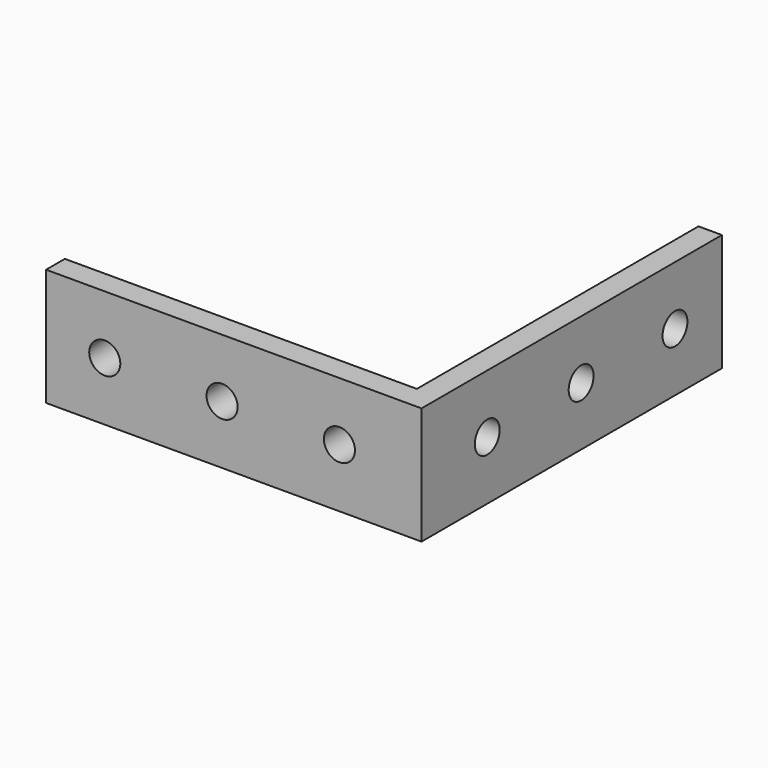
from build123d import *

# Parameters (mm, degrees)
F1_DEPTH  = 20
F2_W      = 9
F2_H      = 20
F2_W_2    = 20
F2_H_2    = 9
F3_DEPTH  = 1.5
F4_W      = 40
F4_H      = 9
F4_W_2    = 9
F4_H_2    = 20
F5_DEPTH  = 1.5
F6_SIZE   = 1.49999
F7_R      = 2.65
F8_DEPTH  = 5.5
F9_R      = 2.65
F10_DEPTH = 5.5


# Not quite as in the source:
# - a fillet or chamfer is up to 0.001 mm smaller than in the source, because OpenCascade refuses the exact size


with BuildPart() as f1:
    # F0 (on Top) → F1 (new body)
    with BuildSketch(Plane.XY):
        Polygon((-64, 0), (0, 0), (0, 64), (-4, 64), (-4, 4), (-64, 4), align=None)
    extrude(amount=F1_DEPTH)

    # F2 (on face) → F3 (join)
    with BuildSketch(Plane(origin=(0, 4, 0), x_dir=(-1, 0, 0), z_dir=(0, 1, 0))):
        with Locations((14, 10)):
            Rectangle(F2_W, F2_H)
        with Locations((34, 10)):
            Rectangle(F2_W, F2_H)
        with Locations((54, 10)):
            Rectangle(F2_W_2, F2_H_2)
    extrude(amount=F3_DEPTH)

    # F4 (on face) → F5 (join)
    with BuildSketch(Plane(origin=(-4, 0, 0), x_dir=(0, -1, 0), z_dir=(-1, 0, 0))):
        with Locations((-44, 10)):
            Rectangle(F4_W, F4_H)
        with Locations((-14, 10)):
            Rectangle(F4_W_2, F4_H_2)
    extrude(amount=F5_DEPTH)

    # F6 (size 1.5 in the source; OpenCascade refuses exactly that, so slightly less here)
    f6_edges = [f1.edges().sort_by_distance(p)[0] for p in [
        (-5.5, 64, 10),
        (-5.5, 44, 14.5),
        (-5.5, 44, 5.5),
        (-5.5, 24, 10),
        (-54, 5.5, 14.5),
        (-54, 5.5, 5.5),
        (-44, 5.5, 10),
        (-64, 5.5, 10),
        (-34, 5.5, 20),
        (-29.5, 5.5, 10),
        (-34, 5.5, 0),
        (-38.5, 5.5, 10),
        (-14, 5.5, 20),
        (-9.5, 5.5, 10),
        (-14, 5.5, 0),
        (-18.5, 5.5, 10),
        (-5.5, 9.5, 10),
        (-5.5, 14, 20),
        (-5.5, 18.5, 10),
        (-5.5, 14, 0),
    ]]
    chamfer(f6_edges, length=F6_SIZE)

    # F7 (on face) → F8 (cut, through all)
    with BuildSketch(Plane(origin=(0, 5.5, 0), x_dir=(-1, 0, 0), z_dir=(0, 1, 0))):
        with Locations((14, 10)):
            Circle(F7_R)
        with Locations((34, 10)):
            Circle(F7_R)
        with Locations((54, 10)):
            Circle(F7_R)
    extrude(amount=-F8_DEPTH, mode=Mode.SUBTRACT)

    # F9 (on face) → F10 (cut, through all)
    with BuildSketch(Plane(origin=(-5.5, 0, 0), x_dir=(0, -1, 0), z_dir=(-1, 0, 0))):
        with Locations((-54, 10)):
            Circle(F9_R)
        with Locations((-34, 10)):
            Circle(F9_R)
        with Locations((-14, 10)):
            Circle(F9_R)
    extrude(amount=-F10_DEPTH, mode=Mode.SUBTRACT)


solid = f1.part
